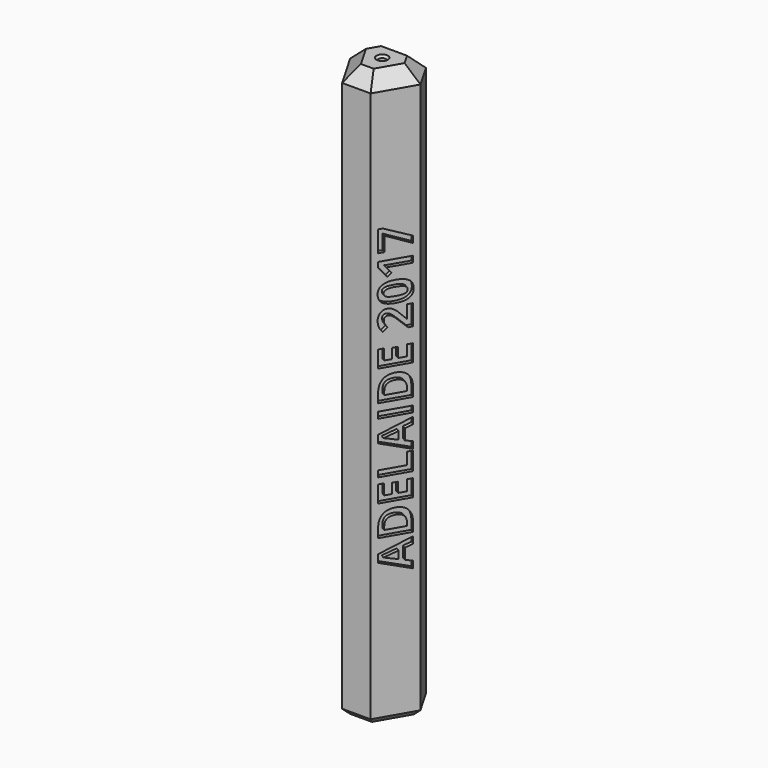
from build123d import *

# Parameters (mm, degrees)
F1_DEPTH        = 63.5
F3_D            = 4.064
F3_DEPTH        = 60.325
F3_CSINK_D      = 4.2672
F3_CSINK_ANGLE  = 90
F3_TIP          = 1.2209487779
F4_SIZE         = 3.175
F5_TEXT_SIZE    = 4.5809615059
F6_DEPTH        = 0.4318
F7_TEXT_SIZE    = 4.5809615059
F8_DEPTH        = 0.4318
F9_TEXT_SIZE    = 4.5809615059
F10_DEPTH       = 0.4318
F12_D           = 0.79375
F12_CSINK_D     = 1.27
F12_CSINK_ANGLE = 90
F13_SIZE        = 0.635
F14_SIZE        = 1.524


# Not quite as in the source:
# - a feature names something its author has since deleted; it is built from what else it names
# - Text() gives the source's letters only with a copy of the font that has no kerning and outlines rounded to 1/6400 em; it was checked with that copy


with BuildPart() as f1:
    # F0 (on Top) → F1 (new body)
    with BuildSketch(Plane.XY):
        Polygon((-5.499261314, 3.175), (0, -6.35), (5.499261314, 3.175), align=None)
    extrude(amount=-F1_DEPTH)

    # F3
    with Locations(Plane(origin=(0, 0, -63.5), x_dir=(1, 0, 0), z_dir=(0, 0, -1))):
        with Locations((0, 0)):
            CounterSinkHole(F3_D / 2, F3_CSINK_D / 2, depth=F3_DEPTH, counter_sink_angle=F3_CSINK_ANGLE)
            with Locations((0, 0, -(F3_DEPTH + F3_TIP / 2))):  # 118° drill point
                Cone(0, F3_D / 2, F3_TIP, mode=Mode.SUBTRACT)

    # F4
    f4_edges = [f1.edges().sort_by_distance(p)[0] for p in [
        (0, -6.35, -31.75),
        (5.499261, 3.175, -31.75),
        (-5.499261, 3.175, -31.75),
    ]]
    chamfer(f4_edges, length=F4_SIZE)

    # F5 (on face) → F6 (cut)
    with BuildSketch(Plane(origin=(0, 3.175, 0), x_dir=(-1, 0, 0), z_dir=(0, 1, 0))):
        with Locations(Location((1.6491461421, -50.8), (0, 0, 90))):
            Text('REYBURN TOOLS', F5_TEXT_SIZE, font='Open Sans', font_style=FontStyle.BOLD, text_align=(TextAlign.LEFT, TextAlign.BOTTOM))
    extrude(amount=-F6_DEPTH, mode=Mode.SUBTRACT)

    # F7 (on face) → F8 (cut)
    with BuildSketch(Plane(origin=(-2.749630657, -1.5875, 0), x_dir=(0.5, -0.8660254038, 0), z_dir=(-0.8660254038, -0.5, 0))):
        with Locations(Location((1.6491461421, -58.2995350279), (0, 0, 90))):
            Text('REYBURN CYBERTUNER', F7_TEXT_SIZE, font='Open Sans', font_style=FontStyle.BOLD, text_align=(TextAlign.LEFT, TextAlign.BOTTOM))
    extrude(amount=-F8_DEPTH, mode=Mode.SUBTRACT)

    # F9 (on face) → F10 (cut)
    with BuildSketch(Plane(origin=(2.749630657, -1.5875, 0), x_dir=(0.5, 0.8660254038, 0), z_dir=(0.8660254038, -0.5, 0))):
        with Locations(Location((1.6491461421, -48.8205235868), (0, 0, 90))):
            Text('ADELAIDE 2017', F9_TEXT_SIZE, font='Open Sans', font_style=FontStyle.BOLD, text_align=(TextAlign.LEFT, TextAlign.BOTTOM))
    extrude(amount=-F10_DEPTH, mode=Mode.SUBTRACT)

    # F12 (through all)
    with Locations(Plane.XY):
        with Locations((0, 0)):
            CounterSinkHole(F12_D / 2, F12_CSINK_D / 2, counter_sink_angle=F12_CSINK_ANGLE)

    # F13
    f13_edges = [f1.edges().sort_by_distance(p)[0] for p in [
        (-2.749631, -1.5875, -63.5),
        (-3.118011, 1.800185, -63.5),
        (0, 3.175, -63.5),
        (3.118011, 1.800185, -63.5),
        (2.749631, -1.5875, -63.5),
        (0, -3.600369, -63.5),
    ]]
    chamfer(f13_edges, length=F13_SIZE)

    # F14
    f14_edges = [f1.edges().sort_by_distance(p)[0] for p in [
        (2.749631, -1.5875, 0),
        (0, -3.600369, 0),
        (-2.749631, -1.5875, 0),
        (-3.118011, 1.800185, 0),
        (0, 3.175, 0),
        (3.118011, 1.800185, 0),
    ]]
    chamfer(f14_edges, length=F14_SIZE)


solid = f1.part
